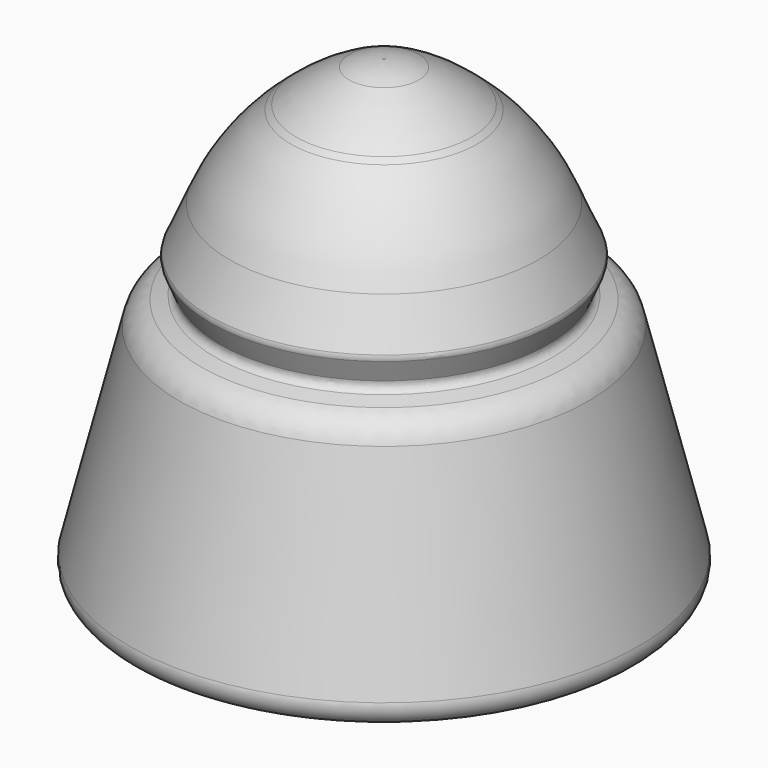
from build123d import *

# Parameters (mm, degrees)
F2_R = 0.2370016828
F3_R = 1.0472005339
F4_R = 7.4210847051
F5_R = 2.7246047928
F6_R = 0.6418579552


with BuildPart() as f1:
    # F0 (on Front) → F1 (revolve)
    with BuildSketch(Plane.XZ):
        Polygon((-8.590772748, 0), (0, 0), (0, 15.1389241219), (-0.5925893784, 15.1389241219), (-2.0398800261, 14.5295374095), (-4.4012479484, 12.5490352511), (-5.7723652571, 9.4259344041), (-5.3153261542, 8.3595104516), (-6.6102705896, 7.978644222), align=None)
    revolve(axis=Axis((0, 0, 7.5694620609), (0, 0, -1)))

    # F2
    f2_edges = [f1.edges().sort_by_distance(p)[0] for p in [
        (5.772365, 0, 9.425934),
        (5.315326, 0, 8.35951),
        (-5.543846, 0, 8.892722),
    ]]
    fillet(f2_edges, radius=F2_R)

    # F3
    f3_edges = [f1.edges().sort_by_distance(p)[0] for p in [
        (6.610271, 0, 7.978644),
    ]]
    fillet(f3_edges, radius=F3_R)

    # F4
    f4_edges = [f1.edges().sort_by_distance(p)[0] for p in [
        (2.03988, 0, 14.529537),
        (4.401248, 0, 12.549035),
        (-3.220564, 0, 13.539286),
    ]]
    fillet(f4_edges, radius=F4_R)

    # F5
    f5_edges = [f1.edges().sort_by_distance(p)[0] for p in [
        (-0.800472, 0, 15.051394),
        (1.008351, 0, 14.963864),
        (0.592589, 0, 15.138924),
    ]]
    fillet(f5_edges, radius=F5_R)

    # F6
    f6_edges = [f1.edges().sort_by_distance(p)[0] for p in [
        (8.590773, 0, 0),
    ]]
    fillet(f6_edges, radius=F6_R)


solid = f1.part
